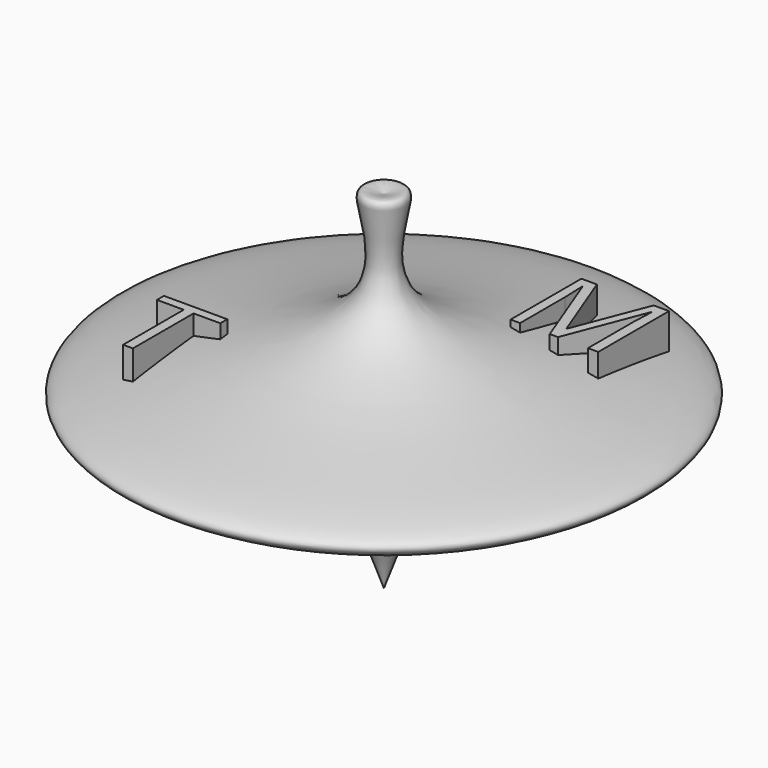
from build123d import *

# Parameters (mm, degrees)
F2_TEXT_SIZE   = 12.4951734001
F2_TEXT_SIZE_2 = 11.9292558843
F3_DEPTH       = 5


# Not quite as in the source:
# - Text() gives the source's letters only with a copy of the font that has no kerning and outlines rounded to 1/6400 em; it was checked with that copy


with BuildPart() as f1:
    # F0 (on Front) → F1 (revolve)
    with BuildSketch(Plane.XZ):
        with BuildLine():
            add(Edge.make_bspline(
                [(0, 17.5), (1.1565975986, 17.825225469), (3.6090819875, 18.5920128312), (-3.9265437359, 3.6317256879), (39.6183643331, 1.2011205052), (10.3663190888, -5.4965580133), (2.622394597, -10.1035475308), (1.2628864497, -13.801545836), (0, -17.5)],
                knots=[0, 0, 0, 0, 0.0749940073, 0.2312656925, 0.4903869105, 0.6939346093, 0.85722893, 1, 1, 1, 1], degree=3))
            Line((0, 17.5), (0, 0))
            Line((0, 0), (0, -17.5))
        make_face()
    revolve(axis=Axis((0, 0, -1.3530924916), (0, 0, -1)))

    # F2 (on Top) → F3 (join)
    with BuildSketch(Plane.XY):
        with Locations((4.9369777553, 8.247400634)):
            Text('M', F2_TEXT_SIZE, font='Open Sans', text_align=(TextAlign.LEFT, TextAlign.BOTTOM))
        with Locations((-17.7662055939, -14.1520593315)):
            Text('T', F2_TEXT_SIZE_2, font='Open Sans', text_align=(TextAlign.LEFT, TextAlign.BOTTOM))
    extrude(amount=F3_DEPTH)


solid = f1.part
